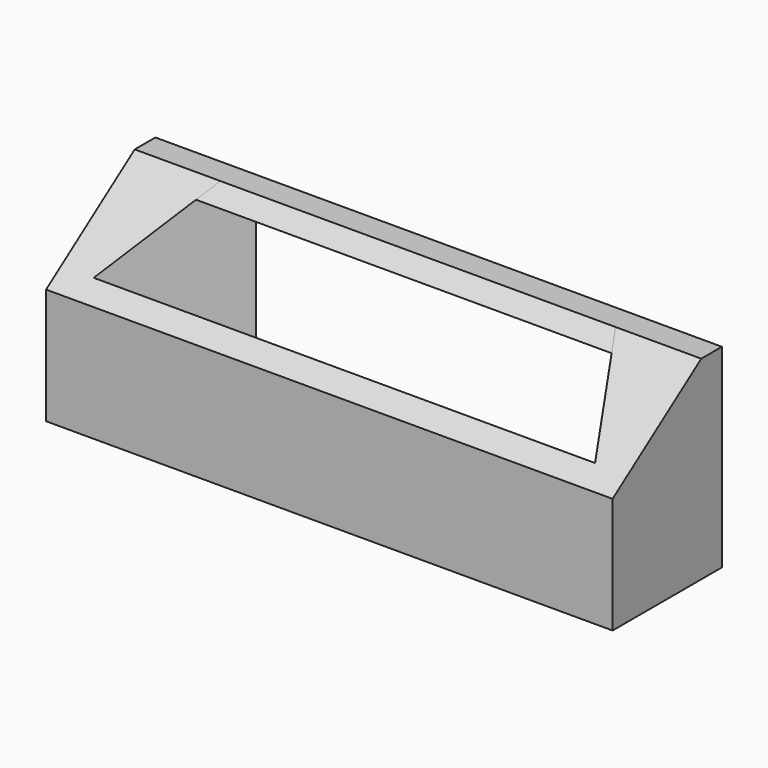
from build123d import *

# Parameters (mm, degrees)
F1_DEPTH    = 56
F2_T1_DEPTH = 363.4104337306
F3_DEPTH    = 56
F6_DEPTH    = 6
F5_W        = 259.5228254795
F5_H        = 121.416632086
F7_DEPTH    = 25
F8_DEPTH    = 52


# Not quite as in the source:
# - a fillet or chamfer that OpenCascade refuses, or shapes differently, is made with other operations: its cross-section is extruded or revolved along the edge and cut away or added


with BuildPart() as f1:
    # F0 (on Top) → F1 (new body)
    with BuildSketch(Plane.XY):
        Polygon((80, -24), (-80, -24), (-58.2867488807, 13.6084541361), (-65.214952111, 13.6084541361), (-73.0717967697, 0), (-90.3923048454, -30), (90.3923048454, -30), (73.0717967697, 0), (65.214952111, 13.6084541361), (58.2867488807, 13.6084541361), align=None)
        Polygon((-90.3923048454, -30), (-73.0717967697, 0), (-90.3923048454, 0), align=None)
        Polygon((90.3923048454, 0), (73.0717967697, 0), (90.3923048454, -30), align=None)
        Polygon((-73.0717967697, 0), (-65.214952111, 13.6084541361), (-90.3923048454, 13.6084541361), (-90.3923048454, 0), align=None)
        Polygon((90.3923048454, 13.6084541361), (65.214952111, 13.6084541361), (73.0717967697, 0), (90.3923048454, 0), align=None)
    extrude(amount=F1_DEPTH)

    # F2: chamfer of 25 x 35.3610857633 on 1 edges, made by hand

    # F2_s2 → F2_t1 (cut)
    with BuildSketch(Plane.YZ.offset(-181.7052168653)):
        Polygon((-30, 31), (5.3610857633, 56), (-30, 56), align=None)
    extrude(amount=F2_T1_DEPTH, mode=Mode.SUBTRACT)

    # F0 (on Top) → F3 (join)
    with BuildSketch(Plane.XY):
        Polygon((-58.2867488807, 13.6084541361), (-80, -24), (80, -24), (58.2867488807, 13.6084541361), align=None)
    extrude(amount=F3_DEPTH)

    # F0 (on Top) → F6 (join)
    with BuildSketch(Plane.XY):
        Polygon((-58.2867488807, 13.6084541361), (-80, -24), (80, -24), (58.2867488807, 13.6084541361), align=None)
        Polygon((80, -24), (-80, -24), (-58.2867488807, 13.6084541361), (-65.214952111, 13.6084541361), (-73.0717967697, 0), (-90.3923048454, -30), (90.3923048454, -30), (73.0717967697, 0), (65.214952111, 13.6084541361), (58.2867488807, 13.6084541361), align=None)
        Polygon((-90.3923048454, -30), (-73.0717967697, 0), (-90.3923048454, 0), align=None)
        Polygon((-73.0717967697, 0), (-65.214952111, 13.6084541361), (-90.3923048454, 13.6084541361), (-90.3923048454, 0), align=None)
        Polygon((90.3923048454, 13.6084541361), (65.214952111, 13.6084541361), (73.0717967697, 0), (90.3923048454, 0), align=None)
        Polygon((90.3923048454, 0), (73.0717967697, 0), (90.3923048454, -30), align=None)
    extrude(amount=-F6_DEPTH)

    # F5 (on offset) → F7 (cut)
    with BuildSketch(Plane(origin=(0, -24.6105813664, 34.8102751353), x_dir=(1, 0, 0), z_dir=(0, -0.5772877121, 0.8165408119))):
        with Locations((5.841344595, -0.7894355804)):
            Rectangle(F5_W, F5_H)
    extrude(amount=F7_DEPTH, mode=Mode.SUBTRACT)

    # F0 (on Top) → F8 (cut)
    with BuildSketch(Plane.XY):
        Polygon((-58.2867488807, 13.6084541361), (-80, -24), (80, -24), (58.2867488807, 13.6084541361), align=None)
    extrude(amount=F8_DEPTH, mode=Mode.SUBTRACT)


solid = f1.part
